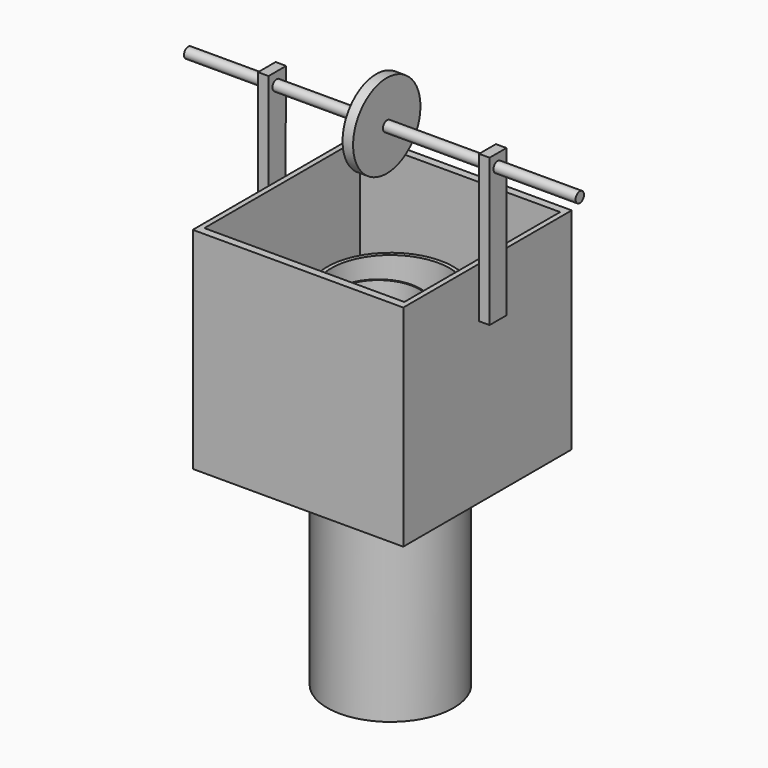
from build123d import *

# Parameters (mm, degrees)
F0_W      = 127
F0_H      = 127
F1_DEPTH  = 127
F2_W      = 120.65
F2_H      = 117.475
F3_DEPTH  = 122.2375
F4_R      = 38.1
F5_DEPTH  = 258.318
F6_R      = 38.1
F7_DEPTH  = 82.55
F9_DEPTH  = 127
F8_R      = 35.71875
F10_DEPTH = 222.25
F11_R     = 35.71875
F12_DEPTH = 181.61
F13_W     = 127
F13_H     = 12.7
F14_DEPTH = 4.7625
F15_W     = 4.7625
F15_H     = 12.7
F16_DEPTH = 3.175
F17_W     = 4.7625
F17_H     = 12.7
F18_DEPTH = 3.175
F21_R     = 59.69
F21_R_2   = 7.493
F22_DEPTH = 1.1938
F24_DEPTH = 50.8
F25_W     = 12.7
F25_H     = 30.48
F25_H_2   = 58.42
F26_DEPTH = 6.35
F27_W     = 12.7
F27_H     = 30.48
F28_DEPTH = 6.35
F29_R     = 3.175
F30_DEPTH = 182.88
F33_R     = 25.4
F34_DEPTH = 3.175


# Not quite as in the source:
# - a feature of the source that left no trace in its solid (it failed there, or was rolled back) is left out
# - a pattern or mirror of a feature is missing from the dataset's text; its kind, count and spacing are read off the source's solid


with BuildPart() as f1:
    # F0 (on Front) → F1 (new body)
    with BuildSketch(Plane.XZ):
        with Locations((63.5, 63.5)):
            Rectangle(F0_W, F0_H)
    extrude(amount=-F1_DEPTH)

    # F2 (on face) → F3 (cut)
    with BuildSketch(Plane.XY.offset(127)):
        with Locations((63.5, 63.5)):
            Rectangle(F2_W, F2_H)
    extrude(amount=-F3_DEPTH, mode=Mode.SUBTRACT)

    # F4 (on face) → F5 (cut)
    with BuildSketch(Plane.XY.offset(127)):
        with Locations((63.5, 69.7174778593)):
            Circle(F4_R)
    extrude(amount=-F5_DEPTH, mode=Mode.SUBTRACT)

    # F11 (on face) → F12 (cut)
    with BuildSketch(Plane.XY.offset(4.7625)):
        with Locations((63.5, 69.7174778593)):
            Circle(F11_R)
    extrude(amount=-F12_DEPTH, mode=Mode.SUBTRACT)

    # F13 (on face) → F14 (cut)
    with BuildSketch(Plane(origin=(0, 127, 0), x_dir=(-1, 0, 0), z_dir=(0, 1, 0))):
        with Locations((-63.5, 31.75)):
            Rectangle(F13_W, F13_H)
    extrude(amount=-F14_DEPTH, mode=Mode.SUBTRACT)

    # F15 (on face) → F16 (join)
    with BuildSketch(Plane.YZ.offset(127)):
        with Locations((124.61875, 31.75)):
            Rectangle(F15_W, F15_H)
    extrude(amount=-F16_DEPTH)

    # F17 (on face) → F18 (join)
    with BuildSketch(Plane(origin=(0, 0, 0), x_dir=(0, -1, 0), z_dir=(-1, 0, 0))):
        with Locations((-124.61875, 31.75)):
            Rectangle(F17_W, F17_H)
    extrude(amount=-F18_DEPTH)

    # F25 (on face) → F26 (join)
    with BuildSketch(Plane.YZ.offset(127)):
        with Locations((63.5, 111.76)):
            Rectangle(F25_W, F25_H)
        with Locations((63.5, 156.21)):
            Rectangle(F25_W, F25_H_2)
    extrude(amount=F26_DEPTH)

    # F27 (on face) → F28 (join)
    with BuildSketch(Plane(origin=(0, 0, 0), x_dir=(0, -1, 0), z_dir=(-1, 0, 0))):
        Polygon((-70.4222992063, 185.42), (-69.85, 127), (-57.15, 127), (-57.15, 185.42), align=None)
        with Locations((-63.5, 111.76)):
            Rectangle(F27_W, F27_H)
    extrude(amount=F28_DEPTH)

    # F29 (on Right) → F30 (join)
    with BuildSketch(Plane.YZ):
        with Locations((63.2532713579, 178.0895883254)):
            Circle(F29_R)
    f30 = extrude(amount=F30_DEPTH)

    # F30_copies: F30 across plane
    add(f30.mirror(Plane(origin=(64.77, 0, 0), x_dir=(0, 0, -1), z_dir=(-1, 0, 0))))

    # F33 (on offset) → F34 (join, symmetric)
    with BuildSketch(Plane.YZ.offset(63.5)):
        with Locations((62.9547689138, 178.3762046341)):
            Circle(F33_R)
    extrude(amount=F34_DEPTH, both=True)


with BuildPart() as f7:
    # F6 (on face) → F7 (new body)
    with BuildSketch(Plane.XY.offset(4.7625)):
        with Locations((63.5, 69.7174778593)):
            Circle(F6_R)
    extrude(amount=F7_DEPTH)


with BuildPart() as f9:
    # F9 (new): a face of the model
    f9_faces = [f7.part.faces().sort_by_distance(p)[0] for p in [
        (63.5, 69.7174778593, 4.7625),
    ]]
    extrude(f9_faces, amount=F9_DEPTH)


with BuildPart() as f10_tool:
    # F8 (on face) → F10 (new body)
    with BuildSketch(Plane.XY.offset(87.3125)):
        with Locations((63.5, 69.7174778593)):
            Circle(F8_R)
    extrude(amount=-F10_DEPTH)


with BuildPart() as f7_1:
    add(f7.part)

    # F10: cut by f10_tool
    add(f10_tool.part, mode=Mode.SUBTRACT)

    # F21 (on plane+point) → F22 (join)
    with BuildSketch(Plane.XY.offset(31.75)):
        with Locations((63.245382659, 108.263690491)):
            Circle(F21_R)
        with Locations((63.245382659, 108.263690491)):
            Circle(F21_R_2, mode=Mode.SUBTRACT)
    extrude(amount=F22_DEPTH)


with BuildPart() as f9_1:
    add(f9.part)

    # F10: cut by f10_tool
    add(f10_tool.part, mode=Mode.SUBTRACT)


with BuildPart() as f24:
    # F23 (on face) → F24 (new body)
    with BuildSketch(Plane.XY.offset(32.9438)):
        with BuildLine():
            ThreePointArc((88.4231645198, 54.143681247), (88.9766971884, 57.1623882847), (89.1621103891, 60.2258197822))
            ThreePointArc((89.1621103891, 60.2258197822), (60.4276466966, 85.4059975394), (39.2375944927, 53.6146080892))
            ThreePointArc((39.2375944927, 53.6146080892), (39.7134324698, 53.4080306163), (40.1910477523, 53.205596245))
            ThreePointArc((40.1910477523, 53.205596245), (60.2149104685, 84.5629499553), (88.3563888363, 60.2258197822))
            ThreePointArc((88.3563888363, 60.2258197822), (88.1359865749, 56.9405964992), (87.4787300717, 53.7142544428))
            ThreePointArc((87.4787300717, 53.7142544428), (87.9518803037, 53.9269158892), (88.4231645198, 54.143681247))
        make_face()
        with BuildLine():
            ThreePointArc((40.1910477523, 53.205596245), (39.7134324698, 53.4080306163), (39.2375944927, 53.6146080892))
            ThreePointArc((39.2375944927, 53.6146080892), (64.0353141115, 34.8272891214), (88.4231645198, 54.143681247))
            ThreePointArc((88.4231645198, 54.143681247), (87.9518803037, 53.9269158892), (87.4787300717, 53.7142544428))
            ThreePointArc((87.4787300717, 53.7142544428), (64.0266477285, 35.6329640648), (40.1910477523, 53.205596245))
        make_face()
    extrude(amount=F24_DEPTH)


solid = Compound([f1.part, f7_1.part, f9_1.part, f24.part])
